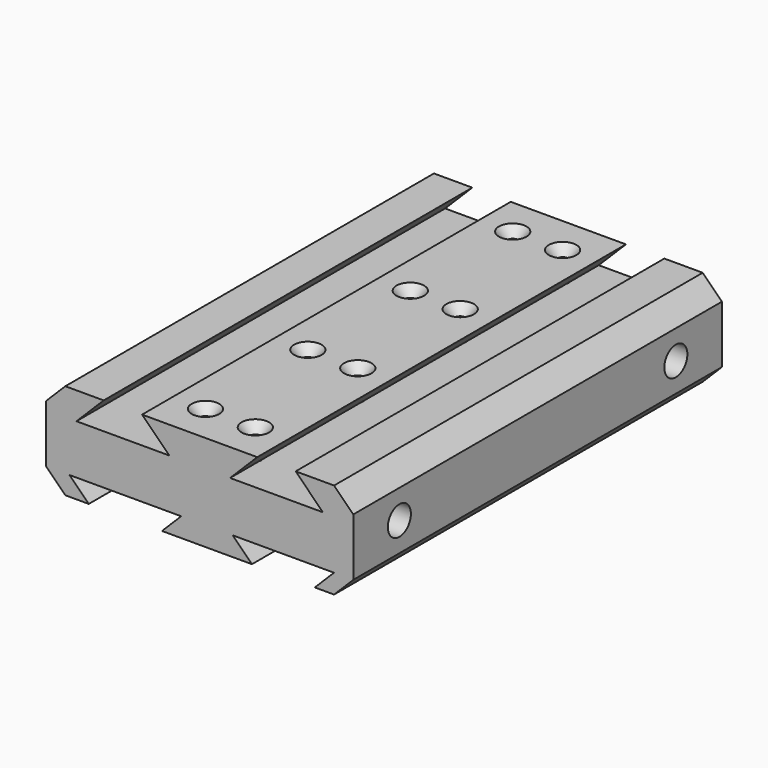
from build123d import *

# Parameters (mm, degrees)
F0_W            = 101.6
F0_H            = 31.75
F1_DEPTH        = 152.4
F3_DEPTH        = 19.05
F5_DEPTH        = 38.1
F7_DEPTH        = 152.401
F8_SIZE         = 6.35
F10_D           = 3.81
F10_DEPTH       = 9.525
F10_CSINK_D     = 9.1186
F10_CSINK_ANGLE = 82
F10_TIP         = 1.1446394792
F12_D           = 6.35
F12_DEPTH       = 25.4
F12_CBORE_D     = 9.525
F12_CBORE_DEPTH = 6.35
F12_TIP         = 1.9077324654
F14_D           = 6.35
F14_DEPTH       = 25.4
F14_CBORE_D     = 9.525
F14_CBORE_DEPTH = 6.35
F14_TIP         = 1.9077324654
F15_TEXT_SIZE   = 8.7312526173
F16_DEPTH       = 3.81


# Not quite as in the source:
# - Text() gives the source's letters only with a copy of the font that has no kerning and outlines rounded to 1/6400 em; it was checked with that copy


with BuildPart() as f1:
    # F0 (on Front) → F1 (new body)
    with BuildSketch(Plane.XZ):
        Rectangle(F0_W, F0_H)
    extrude(amount=F1_DEPTH)

    # F2 (on face) → F3 (cut)
    with BuildSketch(Plane.XZ.offset(152.4)):
        Polygon((44.4238079548, -9.525), (10.9291939616, -9.525), (17.2791939616, -15.875), (38.0738079548, -15.875), align=None)
        Polygon((-6.1240898609, -9.525), (-43.0298241533, -9.525), (-36.6798241533, -15.875), (-12.4740898609, -15.875), align=None)
    extrude(amount=-F3_DEPTH, mode=Mode.SUBTRACT)

    # F4 (on face) → F5 (cut)
    with BuildSketch(Plane(origin=(0, 0, 0), x_dir=(-1, 0, 0), z_dir=(0, 1, 0))):
        Polygon((-4.8768, -9.525), (-45.9232, -9.525), (-39.5732, -15.875), (-11.2268, -15.875), align=None)
        Polygon((39.5732, -15.875), (45.9232, -9.525), (4.8768, -9.525), (11.2268, -15.875), align=None)
    extrude(amount=-F5_DEPTH, mode=Mode.SUBTRACT)

    # F6 (on face) → F7 (cut, through all)
    with BuildSketch(Plane.XZ.offset(152.4)):
        Polygon((-19.05, 15.875), (-31.75, 15.875), (-40.7416, 6.8834), (-10.0584, 6.8834), align=None)
        Polygon((31.75, 15.875), (19.05, 15.875), (10.0584, 6.8834), (40.7416, 6.8834), align=None)
    extrude(amount=-F7_DEPTH, mode=Mode.SUBTRACT)

    # F8
    f8_edges = [f1.edges().sort_by_distance(p)[0] for p in [
        (-50.8, -76.2, 15.875),
        (50.8, -76.2, 15.875),
        (-50.8, -76.2, -15.875),
        (50.8, -76.2, -15.875),
    ]]
    chamfer(f8_edges, length=F8_SIZE)

    # F10
    with Locations(Plane.XY.offset(15.875)):
        with Locations((-8.2549882102, -12.6746), (-8.2549882102, -55.0164), (-8.2549882102, -97.3582), (-8.2549882102, -139.7), (8.2549882102, -139.7), (8.2549882102, -97.3582), (8.2549882102, -55.0164), (8.2549882102, -12.6746)):
            CounterSinkHole(F10_D / 2, F10_CSINK_D / 2, depth=F10_DEPTH, counter_sink_angle=F10_CSINK_ANGLE)
            with Locations((0, 0, -(F10_DEPTH + F10_TIP / 2))):  # 118° drill point
                Cone(0, F10_D / 2, F10_TIP, mode=Mode.SUBTRACT)

    # F12
    with Locations(Plane(origin=(-50.8, 0, 0), x_dir=(0, -1, 0), z_dir=(-1, 0, 0))):
        with Locations((19.05, 0), (133.35, 0)):
            CounterBoreHole(F12_D / 2, F12_CBORE_D / 2, F12_CBORE_DEPTH, depth=F12_DEPTH)
            with Locations((0, 0, -(F12_DEPTH + F12_TIP / 2))):  # 118° drill point
                Cone(0, F12_D / 2, F12_TIP, mode=Mode.SUBTRACT)

    # F14
    with Locations(Plane.YZ.offset(50.8)):
        with Locations((-133.35, 0), (-19.05, 0)):
            CounterBoreHole(F14_D / 2, F14_CBORE_D / 2, F14_CBORE_DEPTH, depth=F14_DEPTH)
            with Locations((0, 0, -(F14_DEPTH + F14_TIP / 2))):  # 118° drill point
                Cone(0, F14_D / 2, F14_TIP, mode=Mode.SUBTRACT)

    # F15 (on face) → F16 (cut)
    with BuildSketch(Plane(origin=(0, 0, -15.875), x_dir=(1, 0, 0), z_dir=(0, 0, -1))):
        with Locations((-40.1478745043, 122.8248775005)):
            Text('Parker Magahey', F15_TEXT_SIZE, font='Open Sans', text_align=(TextAlign.LEFT, TextAlign.BOTTOM))
        with Locations((-40.1478745043, 110.950373941)):
            Text('CTAE Room 711', F15_TEXT_SIZE, font='Open Sans', text_align=(TextAlign.LEFT, TextAlign.BOTTOM))
        with Locations((-40.1478745043, 99.0758703815)):
            Text('GTID: 5590040108', F15_TEXT_SIZE, font='Open Sans', text_align=(TextAlign.LEFT, TextAlign.BOTTOM))
    extrude(amount=-F16_DEPTH, mode=Mode.SUBTRACT)


solid = f1.part
